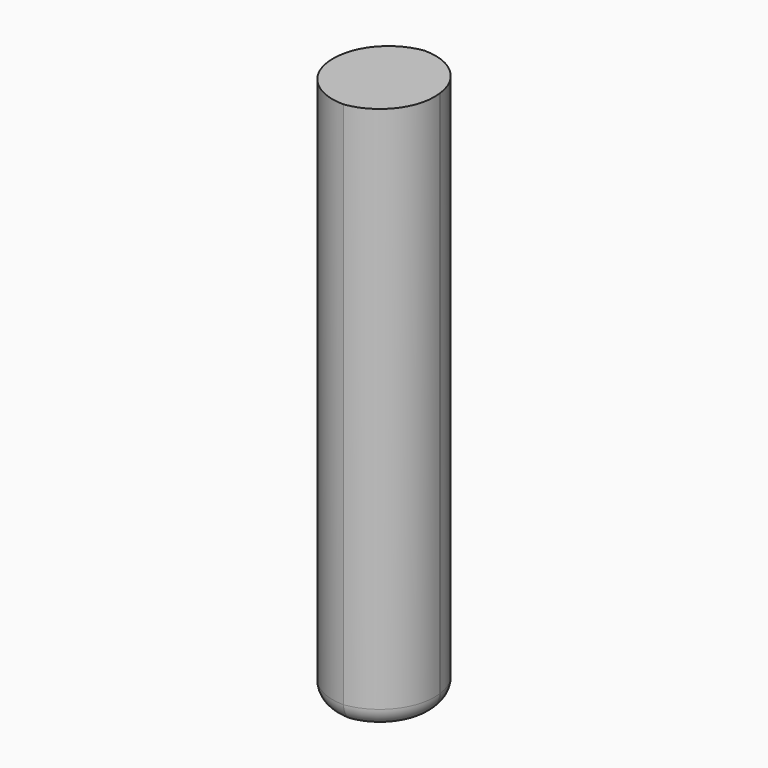
from build123d import *

# Parameters (mm, degrees)
F1_DEPTH     = 15
F2_T1_DEPTH  = 23.0140868267
F2_T3_DEPTH  = 23.0408505773
F2_T5_DEPTH  = 22.0139169115
F2_T7_DEPTH  = 22.0399446
F3_T1_DEPTH  = 0.0435766834
F3_T3_DEPTH  = 0.0435423936
F3_T6_ANGLE  = 137.6611177832
F3_T8_ANGLE  = 137.8590578992
F3_T10_ANGLE = 130.081684858
F3_T12_ANGLE = 130.2935410412


# Not quite as in the source:
# - a fillet or chamfer that OpenCascade refuses, or shapes differently, is made with other operations: its cross-section is extruded or revolved along the edge and cut away or added


with BuildPart() as f1:
    # F0 (on Top) → F1 (new body)
    with BuildSketch(Plane.XY):
        with BuildLine():
            Line((0, -19.5), (0, -22.5))
            ThreePointArc((0, -22.5), (1.5, -22.4499443206), (2.9933259094, -22.3))
            Line((2.9933259094, -22.3), (2.9438857713, -21.9224737536))
            Line((2.9438857713, -21.9224737536), (2.6037776482, -19.3253988247))
            Line((2.6037776482, -19.3253988247), (0, -19.5))
        make_face()
    extrude(amount=-F1_DEPTH)

    # F2: fillet of radius 1.5 on 4 edges, made by hand

    # F2_s2 → F2_t1 (cut)
    with BuildSketch(Plane.XY.offset(-19.0070434133)):
        with BuildLine():
            ThreePointArc((1.3981688146, -22.4565162918), (2.4625908606, -21.9132942034), (2.792258148, -20.7646410751))
            Line((2.792258148, -20.7646410751), (2.9933259094, -22.3))
            ThreePointArc((2.9933259094, -22.3), (2.1971415101, -22.3924667954), (1.3981688146, -22.4565162918))
        make_face()
    extrude(amount=F2_T1_DEPTH, mode=Mode.SUBTRACT)

    # F2_s4 → F2_t3 (cut)
    with BuildSketch(Plane.XY.offset(-19.0204252887)):
        with BuildLine():
            ThreePointArc((1.6071428571, -22.4425286418), (0.4779222842, -22.0442476477), (0, -20.9463600657))
            Line((0, -20.9463600657), (0, -22.5))
            ThreePointArc((0, -22.5), (0.8040850577, -22.4856275701), (1.6071428571, -22.4425286418))
        make_face()
    extrude(amount=F2_T3_DEPTH, mode=Mode.SUBTRACT)

    # F2_s6 → F2_t5 (cut)
    with BuildSketch(Plane.XY.offset(-18.5069584558)):
        with BuildLine():
            ThreePointArc((1.3996400846, -19.4061445189), (0.4044316833, -19.8782200297), (0, -20.9027833823))
            Line((0, -20.9027833823), (0, -19.5))
            Line((0, -19.5), (1.3996400846, -19.4061445189))
        make_face()
    extrude(amount=F2_T5_DEPTH, mode=Mode.SUBTRACT)

    # F2_s8 → F2_t7 (cut)
    with BuildSketch(Plane.XY.offset(-18.5199723)):
        with BuildLine():
            ThreePointArc((1.1989436903, -19.4196025906), (2.2504156143, -19.7563337218), (2.7866041934, -20.7214673234))
            Line((2.7866041934, -20.7214673234), (2.6037776482, -19.3253988247))
            Line((2.6037776482, -19.3253988247), (1.1989436903, -19.4196025906))
        make_face()
    extrude(amount=F2_T7_DEPTH, mode=Mode.SUBTRACT)

    # F3: fillet of radius 0.5 on 6 edges, made by hand

    # F3_s2 → F3_t1 (cut)
    with BuildSketch(Plane.XZ.offset(20.9027833823)):
        with BuildLine():
            ThreePointArc((0, -14.5), (0.1464466094, -14.8535533906), (0.5, -15))
            Line((0.5, -15), (0, -15))
            Line((0, -15), (0, -14.5))
        make_face()
    extrude(amount=F3_T1_DEPTH, mode=Mode.SUBTRACT)

    # F3_s4 → F3_t3 (cut)
    with BuildSketch(Plane(origin=(2.7205290964, -20.7740345789, 0), x_dir=(0, 0, 1), z_dir=(-0.1298494204, 0.9915337251, 0))):
        with BuildLine():
            ThreePointArc((-14.5, 0.0723415147), (-14.8535533906, -0.0741050947), (-15, -0.4276584853))
            Line((-15, -0.4276584853), (-15, 0.0723415147))
            Line((-15, 0.0723415147), (-14.5, 0.0723415147))
        make_face()
    extrude(amount=F3_T3_DEPTH, mode=Mode.SUBTRACT)

    # F3_s5 → F3_t6 (revolve, cut)
    with BuildSketch(Plane(origin=(2.7205290981, -20.7740345786, 0), x_dir=(0, 0, 1), z_dir=(-0.1298494205, 0.9915337251, 0))):
        with BuildLine():
            ThreePointArc((-14.5, 0.072341513), (-14.8535533906, -0.0741050964), (-15, -0.427658487))
            Line((-15, -0.427658487), (-15, 0.072341513))
            Line((-15, 0.072341513), (-14.5, 0.072341513))
        make_face()
    revolve(axis=Axis((1.3049575605, -20.9594152058, -15), (0, 0, -1)), revolution_arc=F3_T6_ANGLE, mode=Mode.SUBTRACT)

    # F3_s7 → F3_t8 (revolve, cut)
    with BuildSketch(Plane(origin=(-9.7457924884, -10.7704005546, 0), x_dir=(0, 0, 1), z_dir=(0.6709566447, 0.7414965819, 0))):
        with BuildLine():
            ThreePointArc((-14.5, 16.6663443409), (-14.8535533906, 16.5198977315), (-15, 16.1663443409))
            Line((-15, 16.1663443409), (-15, 16.6663443409))
            Line((-15, 16.6663443409), (-14.5, 16.6663443409))
        make_face()
    revolve(axis=Axis((1.5000000001, -20.9463600656, -15), (0, 0, -1)), revolution_arc=F3_T8_ANGLE, mode=Mode.SUBTRACT)

    # F3_s9 → F3_t10 (revolve, cut)
    with BuildSketch(Plane.XZ.offset(20.9027833823)):
        with BuildLine():
            ThreePointArc((0, -14.5), (0.1464466094, -14.8535533906), (0.5, -15))
            Line((0.5, -15), (0, -15))
            Line((0, -15), (0, -14.5))
        make_face()
    revolve(axis=Axis((1.5, -20.9027833823, -15), (0, 0, -1)), revolution_arc=F3_T10_ANGLE, mode=Mode.SUBTRACT)

    # F3_s11 → F3_t12 (revolve, cut)
    with BuildSketch(Plane(origin=(-9.8225330213, -10.8154463672, 0), x_dir=(0, 0, 1), z_dir=(-0.672309547, -0.7402701352, 0))):
        with BuildLine():
            ThreePointArc((-14.5, -13.5240244723), (-14.8535533906, -13.6704710817), (-15, -14.0240244723))
            Line((-15, -14.0240244723), (-15, -13.5240244723))
            Line((-15, -13.5240244723), (-14.5, -13.5240244723))
        make_face()
    revolve(axis=Axis((1.2993036057, -20.916241454, -15), (0, 0, -1)), revolution_arc=F3_T12_ANGLE, mode=Mode.SUBTRACT)


solid = f1.part
